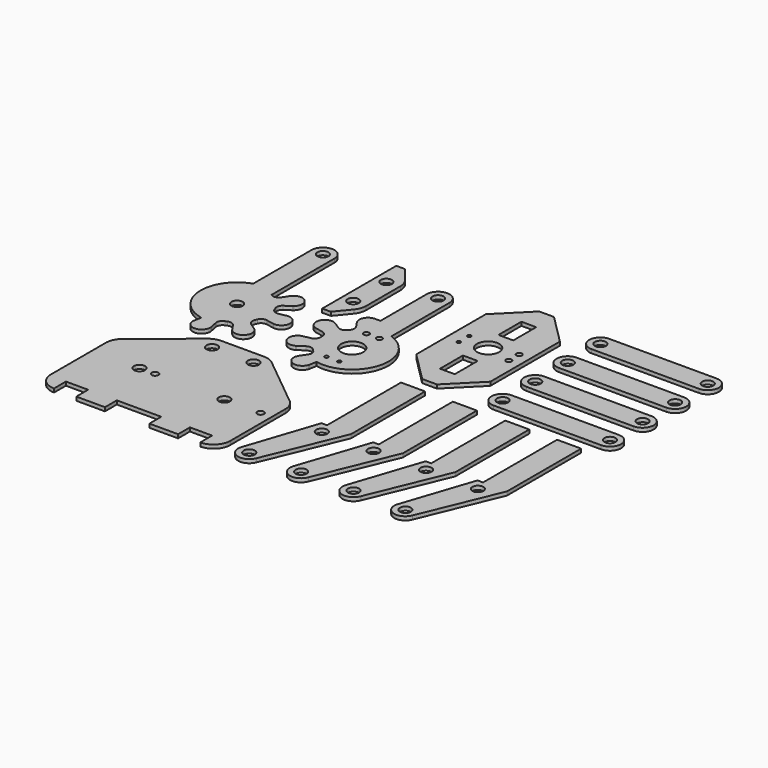
from build123d import *

# Parameters (mm, degrees)
F0_R     = 0.5
F0_R_2   = 3
F0_R_3   = 0.75
F0_R_4   = 1.5
F1_DEPTH = 1
F0_W     = 4
F0_H     = 7.75
F0_R_5   = 0.9


# Not quite as in the source:
# - ends of sketch curves that miss each other by under 0.0002 mm in the source are joined


with BuildPart() as f1:
    # F0 (on Top) → F1 (new body)
    with BuildSketch(Plane.XY):
        with BuildLine():
            Line((-11.705431, 17.401299), (-11.705431, 37.071935))
            ThreePointArc((-11.705431, 37.071935), (-14.810431, 40.176935), (-17.915431, 37.071935))
            Line((-17.915431, 37.071935), (-17.915431, 21.501899))
            Line((-17.915431, 21.501899), (-19.398266, 21.501899))
            ThreePointArc((-19.398266, 21.501899), (-21.4135319513, 20.364414494), (-21.4811508859, 18.0512790601))
            ThreePointArc((-21.4811508859, 18.0512790601), (-21.4740925853, 18.0379767273), (-21.4669493305, 18.0247198206))
            ThreePointArc((-21.4669493305, 18.0247198206), (-21.4125598677, 17.9298705521), (-21.3538246766, 17.8376492167))
            Line((-21.3538246766, 17.8376492167), (-20.2401, 16.175467))
            ThreePointArc((-20.2401, 16.175467), (-19.9849261644, 15.1213822742), (-20.4742852797, 14.1535313003))
            ThreePointArc((-20.4742852797, 14.1535313003), (-20.6868697232, 13.9483732413), (-20.8920277476, 13.7357887649))
            ThreePointArc((-20.8920277476, 13.7357887649), (-21.8598788615, 13.2464302122), (-22.9139629798, 13.5016040301))
            Line((-22.9139629798, 13.5016040301), (-24.576146, 14.615328))
            ThreePointArc((-24.576146, 14.615328), (-24.6683674877, 14.6740634335), (-24.7632170122, 14.7284529775))
            ThreePointArc((-24.7632170122, 14.7284529775), (-24.7764737153, 14.7355961136), (-24.789775843, 14.7426542981))
            ThreePointArc((-24.789775843, 14.7426542981), (-28.0612111654, 13.5605872088), (-26.5838040759, 10.4114857554))
            ThreePointArc((-26.5838040759, 10.4114857554), (-26.569407527, 10.407070735), (-26.5549830297, 10.4027478997))
            ThreePointArc((-26.5549830297, 10.4027478997), (-26.4494548653, 10.3741383085), (-26.3427120231, 10.3504598832))
            Line((-26.3427120231, 10.3504598832), (-24.37985, 9.962641))
            ThreePointArc((-24.37985, 9.962641), (-23.4540642909, 9.3977262573), (-23.1157196127, 8.3673230218))
            ThreePointArc((-23.1157196127, 8.3673230218), (-23.12097, 8.0719345003), (-23.1157187021, 7.7765460106))
            ThreePointArc((-23.1157187021, 7.7765460106), (-23.4540642909, 6.7461427427), (-24.3798499733, 6.181227865))
            Line((-24.3798499733, 6.181227865), (-26.342712, 5.793409))
            ThreePointArc((-26.342712, 5.793409), (-26.4494548653, 5.7697306915), (-26.5549830297, 5.7411211003))
            ThreePointArc((-26.5549830297, 5.7411211003), (-26.569407527, 5.736798265), (-26.5838040759, 5.7323832446))
            ThreePointArc((-26.5838040759, 5.7323832446), (-28.0612111654, 2.5832817912), (-24.789775843, 1.4012147019))
            ThreePointArc((-24.789775843, 1.4012147019), (-24.7764737153, 1.4082728864), (-24.7632170122, 1.4154160225))
            ThreePointArc((-24.7632170122, 1.4154160225), (-24.6683674877, 1.4698055665), (-24.5761459069, 1.528540861))
            Line((-24.5761459069, 1.528540861), (-22.913963, 2.642266))
            ThreePointArc((-22.913963, 2.642266), (-21.8598784981, 2.8974397457), (-20.8920278016, 2.4080801848))
            ThreePointArc((-20.8920278016, 2.4080801848), (-20.6868692235, 2.1954962591), (-20.4742847649, 1.9903382524))
            ThreePointArc((-20.4742847649, 1.9903382524), (-19.9849261644, 1.0224867258), (-20.2401004926, -0.03159767))
            Line((-20.2401004926, -0.03159767), (-21.353825, -1.69378))
            ThreePointArc((-21.353825, -1.69378), (-21.4125598677, -1.7860015521), (-21.4669493305, -1.8808508206))
            ThreePointArc((-21.4669493305, -1.8808508206), (-21.4740925853, -1.8941077273), (-21.4811508859, -1.9074100601))
            ThreePointArc((-21.4811508859, -1.9074100601), (-20.2990840395, -5.1788462355), (-17.1499823846, -3.7014378807))
            ThreePointArc((-17.1499823846, -3.7014378807), (-17.1455673732, -3.6870413335), (-17.1412445468, -3.672616838))
            ThreePointArc((-17.1412445468, -3.672616838), (-17.1126350194, -3.5670886915), (-17.0889566555, -3.4603458705))
            Line((-17.0889566555, -3.4603458705), (-16.716274, -1.574091))
            ThreePointArc((-16.716274, -1.574091), (-5.3038095885, 5.561515595), (-11.705431, 17.401299))
        make_face()
        with Locations((-16.560431, 1.571935)):
            Circle(F0_R, mode=Mode.SUBTRACT)
        with Locations((-14.810431, 8.071935)):
            Circle(F0_R_2, mode=Mode.SUBTRACT)
        with Locations((-13.060431, 1.571935)):
            Circle(F0_R, mode=Mode.SUBTRACT)
        with Locations((-16.560431, 15.071935)):
            Circle(F0_R_3, mode=Mode.SUBTRACT)
        with Locations((-13.060431, 15.071935)):
            Circle(F0_R_3, mode=Mode.SUBTRACT)
        with Locations((-14.810431, 37.071935)):
            Circle(F0_R_4, mode=Mode.SUBTRACT)
    extrude(amount=F1_DEPTH)


with BuildPart() as f1b:
    # F0 (on Top) → F1, piece 2 (new body)
    with BuildSketch(Plane.XY):
        with BuildLine():
            ThreePointArc((-25.526807047, 22.0806820383), (-24.7745553684, 23.4154410904), (-24.513726, 24.92522))
            Line((-24.513726, 24.92522), (-24.513726, 36.491951))
            ThreePointArc((-24.513726, 36.491951), (-24.7745553684, 38.0017299096), (-25.526807047, 39.3364889617))
            Line((-25.526807, 39.336489), (-28.685564, 43.208585))
            Line((-28.685564, 43.208585), (-31.013726, 43.208585))
            Line((-31.013726, 43.208585), (-31.013726, 18.208585))
            Line((-31.013726, 18.208585), (-28.685564, 18.208585))
            Line((-28.685564, 18.208585), (-25.526807, 22.080682))
        make_face()
        with Locations((-28.043726, 24.958585)):
            Circle(F0_R_4, mode=Mode.SUBTRACT)
        with Locations((-28.043726, 36.158585)):
            Circle(F0_R_4, mode=Mode.SUBTRACT)
    extrude(amount=F1_DEPTH)


with BuildPart() as f1c:
    # F0 (on Top) → F1, piece 3 (new body)
    with BuildSketch(Plane.XY):
        with BuildLine():
            ThreePointArc((-42.9306605583, 1.1043160324), (-41.8492135224, 1.1860450069), (-40.9730172163, 0.5469148559))
            Line((-40.9730172163, 0.5469148559), (-39.863564, -1.118122))
            ThreePointArc((-39.863564, -1.118122), (-39.8008392354, -1.2076779553), (-39.7340236566, -1.2942247219))
            ThreePointArc((-39.7340236566, -1.2942247219), (-39.7245097175, -1.3058971218), (-39.7149213035, -1.3175084211))
            ThreePointArc((-39.7149213035, -1.3175084211), (-36.2401515323, -1.4773453759), (-36.3999886787, 1.9974243865))
            ThreePointArc((-36.3999886787, 1.9974243865), (-36.4115999856, 2.0070128056), (-36.423272393, 2.0165267496))
            ThreePointArc((-36.423272393, 2.0165267496), (-36.5098192161, 2.0833423614), (-36.599375324, 2.1460670146))
            Line((-36.599375324, 2.1460670146), (-38.264412, 3.255519))
            ThreePointArc((-38.264412, 3.255519), (-38.9035426924, 4.1317154181), (-38.8218144102, 5.2131627307))
            ThreePointArc((-38.8218144102, 5.2131627307), (-38.7039230905, 5.4840564669), (-38.5957344567, 5.7589691704))
            ThreePointArc((-38.5957344567, 5.7589691704), (-37.8888259406, 6.581458366), (-36.817328185, 6.7490890762))
            Line((-36.817328185, 6.7490890762), (-34.609374, 6.320351))
            ThreePointArc((-34.609374, 6.320351), (-32.039319, 8.6643619541), (-34.6093739465, 11.0083734195))
            Line((-34.6093739465, 11.0083734195), (-36.817328, 10.579635))
            ThreePointArc((-36.817328, 10.579635), (-37.8888258548, 10.7472655862), (-38.595733667, 11.5697551243))
            ThreePointArc((-38.595733667, 11.5697551243), (-38.7039232645, 11.8446679533), (-38.8218151845, 12.1155619158))
            ThreePointArc((-38.8218151845, 12.1155619158), (-38.9035427684, 13.1970093153), (-38.2644121634, 14.0732052452))
            Line((-38.2644121634, 14.0732052452), (-36.599376, 15.182658))
            ThreePointArc((-36.599376, 15.182658), (-36.5098196929, 15.2453822878), (-36.4232728821, 15.3121978544))
            ThreePointArc((-36.4232728821, 15.3121978544), (-36.4116004759, 15.3217117922), (-36.3999891703, 15.3313002049))
            ThreePointArc((-36.3999891703, 15.3313002049), (-36.2401515782, 18.8060704218), (-39.7149217951, 18.6462328297))
            ThreePointArc((-39.7149217951, 18.6462328297), (-39.7245102078, 18.6346215241), (-39.7340241456, 18.6229491179))
            ThreePointArc((-39.7340241456, 18.6229491179), (-39.8008394656, 18.5364026423), (-39.8635638606, 18.4468469071))
            Line((-39.8635638606, 18.4468469071), (-40.973017, 16.78181))
            ThreePointArc((-40.973017, 16.78181), (-41.8492133219, 16.1426790502), (-42.9306609361, 16.2244081401))
            ThreePointArc((-42.9306609361, 16.2244081401), (-43.102918009, 16.3006960609), (-43.2768601529, 16.3730606204))
            Line((-43.2768601529, 16.3730606204), (-43.27686, 37.664362))
            ThreePointArc((-43.27686, 37.664362), (-46.38186, 40.769362), (-49.48686, 37.664362))
            Line((-49.48686, 37.664362), (-49.48686, 17.993726))
            ThreePointArc((-49.48686, 17.993726), (-56.1955728801, 8.0568294852), (-48.3124651136, -0.9767385671))
            Line((-48.3124651136, -0.9767385671), (-48.68999, -2.86203))
            ThreePointArc((-48.68999, -2.86203), (-48.7089626439, -2.9697085902), (-48.7229147042, -3.0781520311))
            ThreePointArc((-48.7229147042, -3.0781520311), (-48.7244409923, -3.0931332679), (-48.7258714111, -3.1081239621))
            ThreePointArc((-48.7258714111, -3.1081239621), (-46.38186, -5.678179), (-44.0378485889, -3.1081239621))
            ThreePointArc((-44.0378485889, -3.1081239621), (-44.0392790077, -3.0931332679), (-44.0408052958, -3.0781520311))
            ThreePointArc((-44.0408052958, -3.0781520311), (-44.0547573561, -2.9697085902), (-44.0737300303, -2.8620300061))
            Line((-44.0737300303, -2.8620300061), (-44.466587, -0.90017))
            ThreePointArc((-44.466587, -0.90017), (-44.2989567373, 0.1713282737), (-43.4764672033, 0.8782365447))
            ThreePointArc((-43.4764672033, 0.8782365447), (-43.2015544669, 0.9864250905), (-42.9306605583, 1.1043160324))
        make_face()
        with Locations((-46.38186, 8.664362)):
            Circle(F0_R_4, mode=Mode.SUBTRACT)
        with Locations((-46.38186, 37.664362)):
            Circle(F0_R_4, mode=Mode.SUBTRACT)
    extrude(amount=F1_DEPTH)


with BuildPart() as f1d:
    # F0 (on Top) → F1, piece 4 (new body)
    with BuildSketch(Plane.XY):
        Polygon((17.543052, 14.264699), (17.543052, 37.764699), (9.543052, 45.764699), (5.543052, 45.764699), (-2.456948, 37.764699), (-2.456948, 14.264699), (5.543052, 6.264699), (9.543052, 6.264699), align=None)
        with Locations((7.543052, 16.139699)):
            Rectangle(F0_W, F0_H, mode=Mode.SUBTRACT)
        with Locations((1.043052, 24.264699)):
            Circle(F0_R, mode=Mode.SUBTRACT)
        with Locations((1.043052, 27.764699)):
            Circle(F0_R, mode=Mode.SUBTRACT)
        with Locations((7.543052, 26.014699)):
            Circle(F0_R_2, mode=Mode.SUBTRACT)
        with Locations((14.543052, 24.264699)):
            Circle(F0_R_3, mode=Mode.SUBTRACT)
        with Locations((14.543052, 27.764699)):
            Circle(F0_R_3, mode=Mode.SUBTRACT)
        with Locations((7.543052, 35.889699)):
            Rectangle(F0_W, F0_H, mode=Mode.SUBTRACT)
    extrude(amount=F1_DEPTH)


with BuildPart() as f1e:
    # F0 (on Top) → F1, piece 5 (new body)
    with BuildSketch(Plane.XY):
        with BuildLine():
            Line((53.902101, 45.227383), (24.902101, 45.227383))
            ThreePointArc((24.902101, 45.227383), (21.902101, 42.227383), (24.902101, 39.227383))
            Line((24.902101, 39.227383), (53.902101, 39.227383))
            ThreePointArc((53.902101, 39.227383), (56.902101, 42.227383), (53.902101, 45.227383))
        make_face()
        with Locations((24.902101, 42.227383)):
            Circle(F0_R_4, mode=Mode.SUBTRACT)
        with Locations((53.902101, 42.227383)):
            Circle(F0_R_4, mode=Mode.SUBTRACT)
    extrude(amount=F1_DEPTH)


with BuildPart() as f1f:
    # F0 (on Top) → F1, piece 6 (new body)
    with BuildSketch(Plane.XY):
        with BuildLine():
            Line((53.902101, 34.227383), (24.902101, 34.227383))
            ThreePointArc((24.902101, 34.227383), (21.902101, 31.227383), (24.902101, 28.227383))
            Line((24.902101, 28.227383), (53.902101, 28.227383))
            ThreePointArc((53.902101, 28.227383), (56.902101, 31.227383), (53.902101, 34.227383))
        make_face()
        with Locations((24.902101, 31.227383)):
            Circle(F0_R_4, mode=Mode.SUBTRACT)
        with Locations((53.902101, 31.227383)):
            Circle(F0_R_4, mode=Mode.SUBTRACT)
    extrude(amount=F1_DEPTH)


with BuildPart() as f1g:
    # F0 (on Top) → F1, piece 7 (new body)
    with BuildSketch(Plane.XY):
        with BuildLine():
            Line((53.902101, 23.227383), (24.902101, 23.227383))
            ThreePointArc((24.902101, 23.227383), (21.902101, 20.227383), (24.902101, 17.227383))
            Line((24.902101, 17.227383), (53.902101, 17.227383))
            ThreePointArc((53.902101, 17.227383), (56.902101, 20.227383), (53.902101, 23.227383))
        make_face()
        with Locations((24.902101, 20.227383)):
            Circle(F0_R_4, mode=Mode.SUBTRACT)
        with Locations((53.902101, 20.227383)):
            Circle(F0_R_4, mode=Mode.SUBTRACT)
    extrude(amount=F1_DEPTH)


with BuildPart() as f1h:
    # F0 (on Top) → F1, piece 8 (new body)
    with BuildSketch(Plane.XY):
        with BuildLine():
            Line((53.902101, 12.227383), (24.902101, 12.227383))
            ThreePointArc((24.902101, 12.227383), (21.902101, 9.227383), (24.902101, 6.227383))
            Line((24.902101, 6.227383), (53.902101, 6.227383))
            ThreePointArc((53.902101, 6.227383), (56.902101, 9.227383), (53.902101, 12.227383))
        make_face()
        with Locations((24.902101, 9.227383)):
            Circle(F0_R_4, mode=Mode.SUBTRACT)
        with Locations((53.902101, 9.227383)):
            Circle(F0_R_4, mode=Mode.SUBTRACT)
    extrude(amount=F1_DEPTH)


with BuildPart() as f1i:
    # F0 (on Top) → F1, piece 9 (new body)
    with BuildSketch(Plane.XY):
        with BuildLine():
            Line((0.874151, -43.825087), (9.567805, -22.794698))
            Line((9.567805, -22.794698), (9.567805, 2.205302))
            Line((9.567805, 2.205302), (3.067805, 2.205302))
            Line((3.067805, 2.205302), (3.067805, -22.794698))
            Line((3.067805, -22.794698), (1.567805, -22.794698))
            Line((1.567805, -22.794698), (-4.800708, -41.886273))
            ThreePointArc((-4.800708, -41.886273), (-2.9021002092, -45.6035857902), (0.874151, -43.825087))
        make_face()
        with Locations((-1.932195, -42.764698)):
            Circle(F0_R_4, mode=Mode.SUBTRACT)
        with Locations((4.067805, -25.794698)):
            Circle(F0_R_4, mode=Mode.SUBTRACT)
    extrude(amount=F1_DEPTH)


with BuildPart() as f1j:
    # F0 (on Top) → F1, piece 10 (new body)
    with BuildSketch(Plane.XY):
        with BuildLine():
            Line((14.874151, -43.825087), (23.567805, -22.794698))
            Line((23.567805, -22.794698), (23.567805, 2.205302))
            Line((23.567805, 2.205302), (17.067805, 2.205302))
            Line((17.067805, 2.205302), (17.067805, -22.794698))
            Line((17.067805, -22.794698), (15.567805, -22.794698))
            Line((15.567805, -22.794698), (9.199292, -41.886273))
            ThreePointArc((9.199292, -41.886273), (11.0978997908, -45.6035857902), (14.874151, -43.825087))
        make_face()
        with Locations((12.067805, -42.764698)):
            Circle(F0_R_4, mode=Mode.SUBTRACT)
        with Locations((18.067805, -25.794698)):
            Circle(F0_R_4, mode=Mode.SUBTRACT)
    extrude(amount=F1_DEPTH)


with BuildPart() as f1k:
    # F0 (on Top) → F1, piece 11 (new body)
    with BuildSketch(Plane.XY):
        with BuildLine():
            Line((28.904246, -43.663975), (37.5979, -22.633586))
            Line((37.5979, -22.633586), (37.5979, 2.366414))
            Line((37.5979, 2.366414), (31.0979, 2.366414))
            Line((31.0979, 2.366414), (31.0979, -22.633586))
            Line((31.0979, -22.633586), (29.5979, -22.633586))
            Line((29.5979, -22.633586), (23.229387, -41.72516))
            ThreePointArc((23.229387, -41.72516), (25.1279943384, -45.4424736356), (28.904246, -43.663975))
        make_face()
        with Locations((26.0979, -42.603586)):
            Circle(F0_R_4, mode=Mode.SUBTRACT)
        with Locations((32.0979, -25.633586)):
            Circle(F0_R_4, mode=Mode.SUBTRACT)
    extrude(amount=F1_DEPTH)


with BuildPart() as f1l:
    # F0 (on Top) → F1, piece 12 (new body)
    with BuildSketch(Plane.XY):
        with BuildLine():
            Line((42.904246, -43.663975), (51.5979, -22.633586))
            Line((51.5979, -22.633586), (51.5979, 2.366414))
            Line((51.5979, 2.366414), (45.0979, 2.366414))
            Line((45.0979, 2.366414), (45.0979, -22.633586))
            Line((45.0979, -22.633586), (43.5979, -22.633586))
            Line((43.5979, -22.633586), (37.229387, -41.72516))
            ThreePointArc((37.229387, -41.72516), (39.1279943384, -45.4424736356), (42.904246, -43.663975))
        make_face()
        with Locations((40.0979, -42.603586)):
            Circle(F0_R_4, mode=Mode.SUBTRACT)
        with Locations((46.0979, -25.633586)):
            Circle(F0_R_4, mode=Mode.SUBTRACT)
    extrude(amount=F1_DEPTH)


with BuildPart() as f1m:
    # F0 (on Top) → F1, piece 13 (new body)
    with BuildSketch(Plane.XY):
        with BuildLine():
            ThreePointArc((-12.9021, -45.603586), (-9.7201194847, -44.2855665153), (-8.4021, -41.103586))
            Line((-8.4021, -41.103586), (-8.4021, -22.467547))
            ThreePointArc((-8.4021, -22.467547), (-8.7446419684, -20.745471881), (-9.7201189847, -19.2855669847))
            Line((-9.7201189847, -19.2855669847), (-24.024196, -7.616668))
            ThreePointArc((-24.024196, -7.616668), (-25.3589554277, -6.8644156044), (-26.868735, -6.603586))
            Line((-26.868735, -6.603586), (-38.435465, -6.603586))
            ThreePointArc((-38.435465, -6.603586), (-39.9452445723, -6.8644156044), (-41.2800040519, -7.6166679364))
            Line((-41.2800040519, -7.6166679364), (-55.58408, -19.285567))
            ThreePointArc((-55.58408, -19.285567), (-56.5595578963, -20.7454715544), (-56.9021, -22.467547))
            Line((-56.9021, -22.467547), (-56.9021, -41.103586))
            ThreePointArc((-56.9021, -41.103586), (-55.5840805153, -44.2855665153), (-52.4021, -45.603586))
            Line((-52.4021, -45.603586), (-52.4021, -41.603586))
            Line((-52.4021, -41.603586), (-46.4021, -41.603586))
            Line((-46.4021, -41.603586), (-46.4021, -45.603586))
            Line((-46.4021, -45.603586), (-38.6521, -45.603586))
            Line((-38.6521, -45.603586), (-38.6521, -41.603586))
            Line((-38.6521, -41.603586), (-26.6521, -41.603586))
            Line((-26.6521, -41.603586), (-26.6521, -45.603586))
            Line((-26.6521, -45.603586), (-18.9021, -45.603586))
            Line((-18.9021, -45.603586), (-18.9021, -41.603586))
            Line((-18.9021, -41.603586), (-12.9021, -41.603586))
            Line((-12.9021, -41.603586), (-12.9021, -45.603586))
        make_face()
        with Locations((-44.1021, -27.103586)):
            Circle(F0_R_4, mode=Mode.SUBTRACT)
        with Locations((-39.9021, -27.103586)):
            Circle(F0_R_5, mode=Mode.SUBTRACT)
        with Locations((-21.2021, -27.103586)):
            Circle(F0_R_4, mode=Mode.SUBTRACT)
        with Locations((-11.4021, -27.103586)):
            Circle(F0_R_5, mode=Mode.SUBTRACT)
        with Locations((-38.1021, -10.133586)):
            Circle(F0_R_4, mode=Mode.SUBTRACT)
        with Locations((-26.9021, -10.133586)):
            Circle(F0_R_4, mode=Mode.SUBTRACT)
    extrude(amount=F1_DEPTH)


solid = Compound([f1.part, f1b.part, f1c.part, f1d.part, f1e.part, f1f.part, f1g.part, f1h.part, f1i.part, f1j.part, f1k.part, f1l.part, f1m.part])
